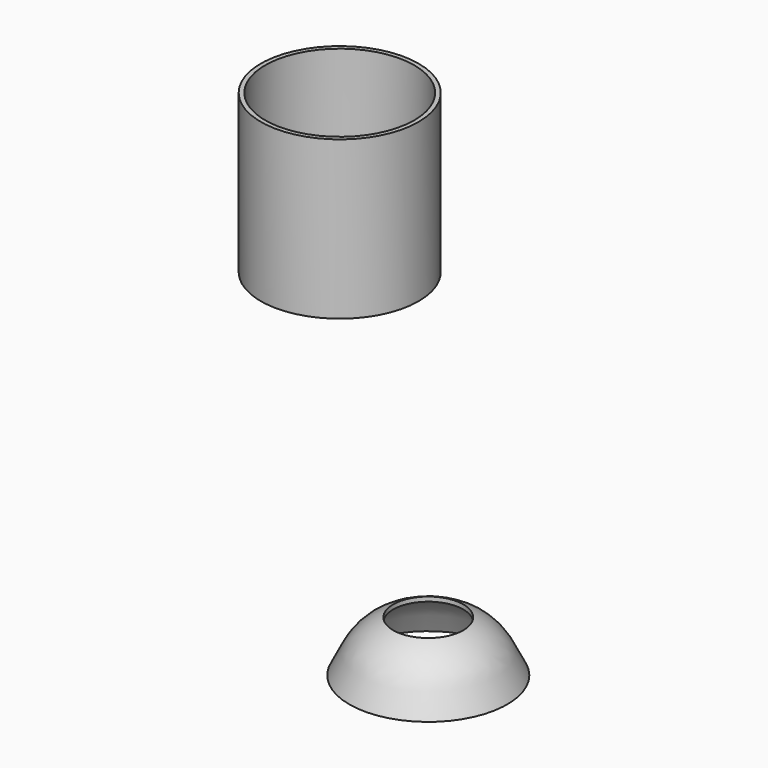
from build123d import *

# Parameters (mm, degrees)
F0_R     = 9
F0_R_2   = 8.5
F1_DEPTH = 18


with BuildPart() as f1:
    # F0 (on Top) → F1 (new body)
    with BuildSketch(Plane.XY):
        with Locations((-54.7211095691, 55.7828843594)):
            Circle(F0_R)
        with Locations((-54.7211095691, 55.7828843594)):
            Circle(F0_R_2, mode=Mode.SUBTRACT)
    extrude(amount=F1_DEPTH)


with BuildPart() as f3:
    # F2 (on Front) → F3 (revolve)
    with BuildSketch(Plane.XZ):
        with BuildLine():
            add(Edge.make_bspline(
                [(-9, 0), (-8.2061928864, 1.756192534), (-7.0883196397, 4.2293381157), (-4.7437136695, 5.5088051811), (-4, 5.8174179779)],
                knots=[0, 0, 0, 0, 0.4814110146, 0.6779436063, 0.6779436063, 0.6779436063, 0.6779436063], degree=3))
            Line((-9, 0), (-8.5, 0))
            add(Edge.make_bspline(
                [(-8.5, 0), (-7.7234594348, 1.643246113), (-6.6733334202, 3.8654302064), (-4.5898606377, 5.0451498847), (-4, 5.30502297)],
                knots=[0, 0, 0, 0, 0.4829129871, 0.6530499844, 0.6530499844, 0.6530499844, 0.6530499844], degree=3))
            Line((-4, 5.30502297), (-4, 5.3174179779))
            Line((-4, 5.3174179779), (-4, 5.8174179779))
        make_face()
    revolve(axis=Axis((0, 0, 3.5), (0, 0, 1)))


solid = Compound([f1.part, f3.part])
